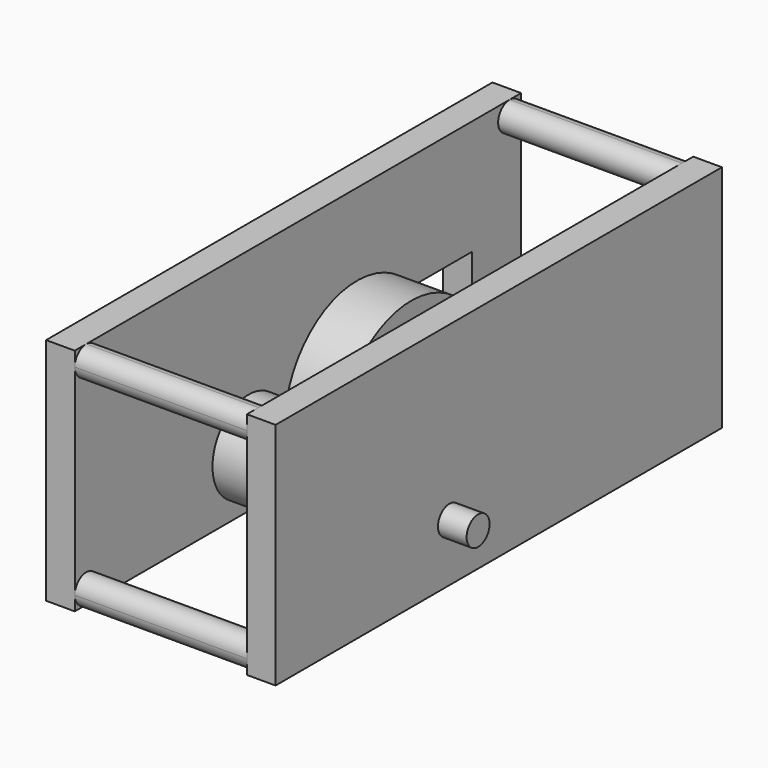
from build123d import *

# Parameters (mm, degrees)
F0_R      = 5
F0_R_2    = 1.8415
F0_R_3    = 1.5875
F1_DEPTH  = 3.175
F2_DEPTH  = 19.05
F3_R      = 1.7145
F4_DEPTH  = 3.175
F3_R_2    = 1.5875
F5_DEPTH  = 3.175
F6_DEPTH  = 6
F3_R_3    = 1.8415
F7_DEPTH  = 6
F8_DEPTH  = 3.175
F9_DEPTH  = 25.4
F10_DEPTH = 6


# Not quite as in the source:
# - a feature names something its author has since deleted; it is built from what else it names


with BuildPart() as f1:
    # F0 (on Right) → F1 (new body)
    with BuildSketch(Plane.YZ):
        with BuildLine():
            ThreePointArc((18.4078367749, 6.35), (25.0352423421, 15.7641174197), (36.1329581332, 12.7))
            Line((36.1329581332, 12.7), (44.2828367749, 12.7))
            Line((44.2828367749, 12.7), (44.2828367749, 0))
            Line((44.2828367749, 0), (49.5203367749, 0))
            ThreePointArc((49.5203367749, 0), (48.3978047598, 2.7100320151), (51.1078367749, 1.5875))
            Line((51.1078367749, 1.5875), (51.1078367749, 23.8125))
            ThreePointArc((51.1078367749, 23.8125), (48.3978047598, 22.6899679849), (49.5203367749, 25.4))
            Line((49.5203367749, 25.4), (41.8216693056, 25.4))
            Line((41.8216693056, 25.4), (35.8211970083, 25.4))
            Line((35.8211970083, 25.4), (-9.0546632251, 25.4))
            ThreePointArc((-9.0546632251, 25.4), (-7.9321312099, 24.9350320151), (-7.4671632251, 23.8125))
            ThreePointArc((-7.4671632251, 23.8125), (-9.0546632251, 22.225), (-10.6421632251, 23.8125))
            Line((-10.6421632251, 23.8125), (-10.6421632251, 1.5875))
            ThreePointArc((-10.6421632251, 1.5875), (-9.0546632251, 3.175), (-7.4671632251, 1.5875))
            ThreePointArc((-7.4671632251, 1.5875), (-7.9321312099, 0.4649679849), (-9.0546632251, 0))
            Line((-9.0546632251, 0), (20.6827154167, 0))
            ThreePointArc((20.6827154167, 0), (18.9937193553, 2.9774055671), (18.4078367749, 6.35))
        make_face()
        with Locations((13.4078367749, 6.35)):
            Circle(F0_R, mode=Mode.SUBTRACT)
        with BuildLine():
            ThreePointArc((36.1329581332, 0), (37.8219541946, 2.9774055671), (38.4078367749, 6.35))
            ThreePointArc((38.4078367749, 6.35), (37.8219541946, 9.7225944329), (36.1329581332, 12.7))
            Line((36.1329581332, 12.7), (22.0578367749, 12.7))
            Line((22.0578367749, 12.7), (22.0578367749, 0))
            Line((22.0578367749, 0), (36.1329581332, 0))
        make_face()
        with Locations((28.4078367749, 6.35)):
            Circle(F0_R_2, mode=Mode.SUBTRACT)
        with BuildLine():
            ThreePointArc((36.1329581332, 12.7), (37.8219541946, 9.7225944329), (38.4078367749, 6.35))
            ThreePointArc((38.4078367749, 6.35), (37.8219541946, 2.9774055671), (36.1329581332, 0))
            Line((36.1329581332, 0), (43.4878367749, 0))
            Line((43.4878367749, 0), (44.2828367749, 0))
            Line((44.2828367749, 0), (44.2828367749, 12.7))
            Line((44.2828367749, 12.7), (36.1329581332, 12.7))
        make_face()
        with Locations((13.4078367749, 6.35)):
            Circle(F0_R)
        with Locations((13.4078367749, 6.35)):
            Circle(F0_R_3, mode=Mode.SUBTRACT)
        with BuildLine():
            Line((22.0578367749, 12.7), (36.1329581332, 12.7))
            ThreePointArc((36.1329581332, 12.7), (25.0352423421, 15.7641174197), (18.4078367749, 6.35))
            ThreePointArc((18.4078367749, 6.35), (18.9937193553, 2.9774055671), (20.6827154167, 0))
            Line((20.6827154167, 0), (22.0578367749, 0))
            Line((22.0578367749, 0), (22.0578367749, 12.7))
        make_face()
        with Locations((28.4078367749, 6.35)):
            Circle(F0_R_2)
        with Locations((28.4078367749, 6.35)):
            Circle(F0_R_3, mode=Mode.SUBTRACT)
        with BuildLine():
            ThreePointArc((-10.6421632251, 1.5875), (-10.1771952402, 0.4649679849), (-9.0546632251, 0))
            ThreePointArc((-9.0546632251, 0), (-7.9321312099, 0.4649679849), (-7.4671632251, 1.5875))
            ThreePointArc((-7.4671632251, 1.5875), (-9.0546632251, 3.175), (-10.6421632251, 1.5875))
        make_face()
        with BuildLine():
            ThreePointArc((51.1078367749, 1.5875), (48.3978047598, 2.7100320151), (49.5203367749, 0))
            ThreePointArc((49.5203367749, 0), (50.6428687901, 0.4649679849), (51.1078367749, 1.5875))
        make_face()
        with BuildLine():
            ThreePointArc((-9.0546632251, 25.4), (-10.1771952402, 24.9350320151), (-10.6421632251, 23.8125))
            ThreePointArc((-10.6421632251, 23.8125), (-9.0546632251, 22.225), (-7.4671632251, 23.8125))
            ThreePointArc((-7.4671632251, 23.8125), (-7.9321312099, 24.9350320151), (-9.0546632251, 25.4))
        make_face()
        with BuildLine():
            ThreePointArc((49.5203367749, 25.4), (48.3978047598, 22.6899679849), (51.1078367749, 23.8125))
            ThreePointArc((51.1078367749, 23.8125), (50.6428687901, 24.9350320151), (49.5203367749, 25.4))
        make_face()
        with Locations((28.4078367749, 6.35)):
            Circle(F0_R_3)
        with BuildLine():
            Line((-10.6421632251, 0), (-9.0546632251, 0))
            ThreePointArc((-9.0546632251, 0), (-10.1771952402, 0.4649679849), (-10.6421632251, 1.5875))
            Line((-10.6421632251, 1.5875), (-10.6421632251, 0))
        make_face()
        with BuildLine():
            ThreePointArc((51.1078367749, 1.5875), (50.6428687901, 0.4649679849), (49.5203367749, 0))
            Line((49.5203367749, 0), (50.2833090723, 0))
            Line((50.2833090723, 0), (51.1078367749, 0))
            Line((51.1078367749, 0), (51.1078367749, 1.5875))
        make_face()
        with BuildLine():
            Line((-10.6421632251, 25.4), (-10.6421632251, 23.8125))
            ThreePointArc((-10.6421632251, 23.8125), (-10.1771952402, 24.9350320151), (-9.0546632251, 25.4))
            Line((-9.0546632251, 25.4), (-10.6421632251, 25.4))
        make_face()
        with BuildLine():
            ThreePointArc((49.5203367749, 25.4), (50.6428687901, 24.9350320151), (51.1078367749, 23.8125))
            Line((51.1078367749, 23.8125), (51.1078367749, 25.4))
            Line((51.1078367749, 25.4), (49.5203367749, 25.4))
        make_face()
    extrude(amount=F1_DEPTH)


with BuildPart() as f2:
    # F0 (on Right) → F2 (new body)
    with BuildSketch(Plane.YZ):
        with BuildLine():
            ThreePointArc((-10.6421632251, 1.5875), (-10.1771952402, 0.4649679849), (-9.0546632251, 0))
            ThreePointArc((-9.0546632251, 0), (-7.9321312099, 0.4649679849), (-7.4671632251, 1.5875))
            ThreePointArc((-7.4671632251, 1.5875), (-9.0546632251, 3.175), (-10.6421632251, 1.5875))
        make_face()
    extrude(amount=-F2_DEPTH)


with BuildPart() as f2b:
    # F0 (on Right) → F2, piece 2 (new body)
    with BuildSketch(Plane.YZ):
        with BuildLine():
            ThreePointArc((51.1078367749, 1.5875), (48.3978047598, 2.7100320151), (49.5203367749, 0))
            ThreePointArc((49.5203367749, 0), (50.6428687901, 0.4649679849), (51.1078367749, 1.5875))
        make_face()
    extrude(amount=-F2_DEPTH)


with BuildPart() as f2c:
    # F0 (on Right) → F2, piece 3 (new body)
    with BuildSketch(Plane.YZ):
        with BuildLine():
            ThreePointArc((-9.0546632251, 25.4), (-10.1771952402, 24.9350320151), (-10.6421632251, 23.8125))
            ThreePointArc((-10.6421632251, 23.8125), (-9.0546632251, 22.225), (-7.4671632251, 23.8125))
            ThreePointArc((-7.4671632251, 23.8125), (-7.9321312099, 24.9350320151), (-9.0546632251, 25.4))
        make_face()
    extrude(amount=-F2_DEPTH)


with BuildPart() as f2d:
    # F0 (on Right) → F2, piece 4 (new body)
    with BuildSketch(Plane.YZ):
        with BuildLine():
            ThreePointArc((49.5203367749, 25.4), (48.3978047598, 22.6899679849), (51.1078367749, 23.8125))
            ThreePointArc((51.1078367749, 23.8125), (50.6428687901, 24.9350320151), (49.5203367749, 25.4))
        make_face()
    extrude(amount=-F2_DEPTH)


with BuildPart() as f4:
    # F3 (on face) → F4 (new body)
    with BuildSketch(Plane(origin=(-19.05, 0, 0), x_dir=(0, -1, 0), z_dir=(-1, 0, 0))):
        with BuildLine():
            Line((10.6421632251, 25.4), (-49.5203367749, 25.4))
            ThreePointArc((-49.5203367749, 25.4), (-48.3978047598, 24.9350320151), (-47.9328367749, 23.8125))
            ThreePointArc((-47.9328367749, 23.8125), (-49.5203367749, 22.225), (-51.1078367749, 23.8125))
            Line((-51.1078367749, 23.8125), (-51.1078367749, 0))
            Line((-51.1078367749, 0), (-44.2828367749, 0))
            Line((-44.2828367749, 0), (-44.2828367749, 12.7))
            Line((-44.2828367749, 12.7), (-36.1329581332, 12.7))
            ThreePointArc((-36.1329581332, 12.7), (-25.0352423421, 15.7641174197), (-18.4078367749, 6.35))
            ThreePointArc((-18.4078367749, 6.35), (-18.9937193553, 2.9774055671), (-20.6827154167, 0))
            Line((-20.6827154167, 0), (10.6421632251, 0))
            Line((10.6421632251, 0), (10.6421632251, 25.4))
        make_face()
        with BuildLine():
            ThreePointArc((-8.4078367749, 6.35), (-13.4078367749, 1.35), (-18.4078367749, 6.35))
            ThreePointArc((-18.4078367749, 6.35), (-13.4078367749, 11.35), (-8.4078367749, 6.35))
        make_face(mode=Mode.SUBTRACT)
        with BuildLine():
            ThreePointArc((-8.4078367749, 6.35), (-13.4078367749, 11.35), (-18.4078367749, 6.35))
            ThreePointArc((-18.4078367749, 6.35), (-13.4078367749, 1.35), (-8.4078367749, 6.35))
        make_face()
        with Locations((-13.4078367749, 6.35)):
            Circle(F3_R, mode=Mode.SUBTRACT)
        with BuildLine():
            Line((-22.0578367749, 0), (-20.6827154167, 0))
            ThreePointArc((-20.6827154167, 0), (-18.9937193553, 2.9774055671), (-18.4078367749, 6.35))
            ThreePointArc((-18.4078367749, 6.35), (-25.0352423421, 15.7641174197), (-36.1329581332, 12.7))
            Line((-36.1329581332, 12.7), (-22.0578367749, 12.7))
            Line((-22.0578367749, 12.7), (-22.0578367749, 6.35))
            Line((-22.0578367749, 6.35), (-22.0578367749, 0))
        make_face()
        with BuildLine():
            ThreePointArc((-47.9328367749, 23.8125), (-48.3978047598, 24.9350320151), (-49.5203367749, 25.4))
            ThreePointArc((-49.5203367749, 25.4), (-50.6428687901, 24.9350320151), (-51.1078367749, 23.8125))
            ThreePointArc((-51.1078367749, 23.8125), (-49.5203367749, 22.225), (-47.9328367749, 23.8125))
        make_face()
        with BuildLine():
            Line((-49.5203367749, 25.4), (-51.1078367749, 25.4))
            Line((-51.1078367749, 25.4), (-51.1078367749, 23.8125))
            ThreePointArc((-51.1078367749, 23.8125), (-50.6428687901, 24.9350320151), (-49.5203367749, 25.4))
        make_face()
    extrude(amount=F4_DEPTH)


with BuildPart() as f5:
    # F3 (on face) → F5 (new body)
    with BuildSketch(Plane(origin=(-19.05, 0, 0), x_dir=(0, -1, 0), z_dir=(-1, 0, 0))):
        with Locations((-28.4078367749, 6.35)):
            Circle(F3_R_2)
    extrude(amount=F5_DEPTH)

    # F3 (on face) → F6 (join)
    with BuildSketch(Plane(origin=(-19.05, 0, 0), x_dir=(0, -1, 0), z_dir=(-1, 0, 0))):
        with Locations((-28.4078367749, 6.35)):
            Circle(F3_R_2)
    extrude(amount=-F6_DEPTH)


with BuildPart() as f7:
    # F3 (on face) → F7 (new body)
    with BuildSketch(Plane(origin=(-19.05, 0, 0), x_dir=(0, -1, 0), z_dir=(-1, 0, 0))):
        with BuildLine():
            ThreePointArc((-36.1329581332, 12.7), (-38.4078367749, 6.35), (-36.1329581332, 0))
            Line((-36.1329581332, 0), (-22.0578367749, 0))
            Line((-22.0578367749, 0), (-22.0578367749, 6.35))
            Line((-22.0578367749, 6.35), (-22.0578367749, 12.7))
            Line((-22.0578367749, 12.7), (-36.1329581332, 12.7))
        make_face()
        with Locations((-28.4078367749, 6.35)):
            Circle(F3_R_3, mode=Mode.SUBTRACT)
        with BuildLine():
            Line((-22.0578367749, 0), (-20.6827154167, 0))
            ThreePointArc((-20.6827154167, 0), (-18.9937193553, 2.9774055671), (-18.4078367749, 6.35))
            ThreePointArc((-18.4078367749, 6.35), (-25.0352423421, 15.7641174197), (-36.1329581332, 12.7))
            Line((-36.1329581332, 12.7), (-22.0578367749, 12.7))
            Line((-22.0578367749, 12.7), (-22.0578367749, 6.35))
            Line((-22.0578367749, 6.35), (-22.0578367749, 0))
        make_face()
        with BuildLine():
            ThreePointArc((-36.1329581332, 0), (-28.4078367749, -3.65), (-20.6827154167, 0))
            Line((-20.6827154167, 0), (-22.0578367749, 0))
            Line((-22.0578367749, 0), (-36.1329581332, 0))
        make_face()
        with Locations((-28.4078367749, 6.35)):
            Circle(F3_R_3)
        with Locations((-28.4078367749, 6.35)):
            Circle(F3_R_2, mode=Mode.SUBTRACT)
    extrude(amount=-F7_DEPTH)


with BuildPart() as f8:
    # F3 (on face) → F8 (new body)
    with BuildSketch(Plane(origin=(-19.05, 0, 0), x_dir=(0, -1, 0), z_dir=(-1, 0, 0))):
        with Locations((-13.4078367749, 6.35)):
            Circle(F3_R_2)
    extrude(amount=F8_DEPTH)

    # F3 (on face) → F9 (join)
    with BuildSketch(Plane(origin=(-19.05, 0, 0), x_dir=(0, -1, 0), z_dir=(-1, 0, 0))):
        with Locations((-13.4078367749, 6.35)):
            Circle(F3_R_2)
    extrude(amount=-F9_DEPTH)


with BuildPart() as f10:
    # F3 (on face) → F10 (new body)
    with BuildSketch(Plane(origin=(-19.05, 0, 0), x_dir=(0, -1, 0), z_dir=(-1, 0, 0))):
        with BuildLine():
            ThreePointArc((-8.4078367749, 6.35), (-13.4078367749, 11.35), (-18.4078367749, 6.35))
            ThreePointArc((-18.4078367749, 6.35), (-13.4078367749, 1.35), (-8.4078367749, 6.35))
        make_face()
        with Locations((-13.4078367749, 6.35)):
            Circle(F3_R, mode=Mode.SUBTRACT)
        with Locations((-13.4078367749, 6.35)):
            Circle(F3_R)
        with Locations((-13.4078367749, 6.35)):
            Circle(F3_R_2, mode=Mode.SUBTRACT)
    extrude(amount=-F10_DEPTH)


solid = Compound([f1.part, f2.part, f2b.part, f2c.part, f2d.part, f4.part, f5.part, f7.part, f8.part, f10.part])
